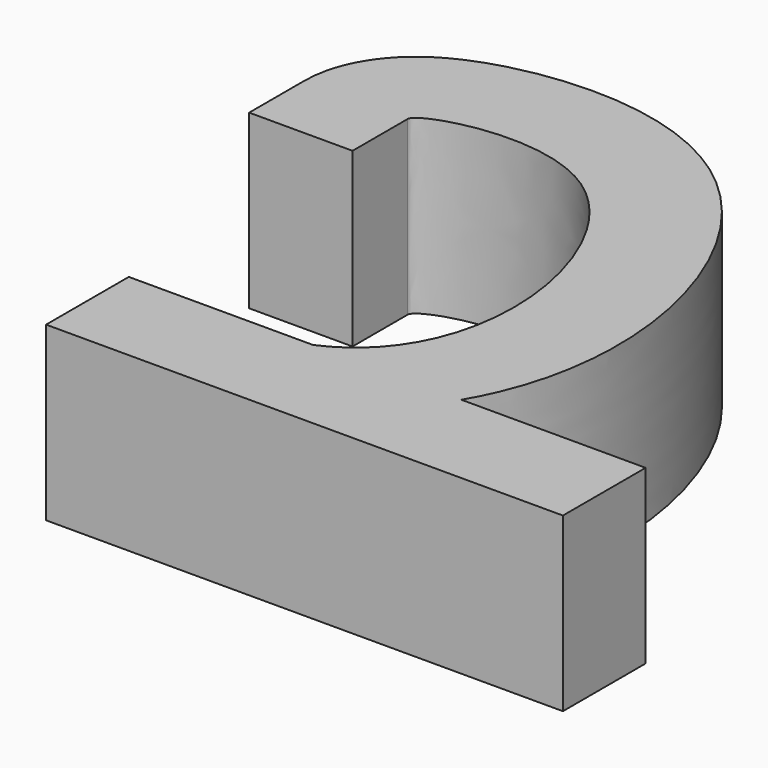
from build123d import *

# Parameters (mm, degrees)
F0_W     = 3
F0_H     = 2
F1_DEPTH = 5


# Not quite as in the source:
# - ends of sketch curves that miss each other by under 0.0002 mm in the source are joined
# - the dataset's text gives a spline's control points without its knots; the knots are read off the source's solid


with BuildPart() as f1:
    # F0 (on Top) → F1 (new body)
    with BuildSketch(Plane.XY):
        Polygon((0.2503667564, 0), (-5.0978784384, 0), (-5.0978784384, -3), (9.9021215616, -3), (9.9021215616, 0), (4.5538399041, 0), align=None)
        with BuildLine():
            add(Edge.make_bspline(
                [(-5.0038373292, 10), (-5.0038373292, 10.4105466628), (2.1157200772, 12.6615455049), (4.0203314378, 1.6529998477), (0.2503667564, 0)],
                knots=[0, 0, 0, 0, 0.4142686249, 1, 1, 1, 1], degree=3))
            Line((0.2503667564, 0), (4.5538399041, 0))
            add(Edge.make_bspline(
                [(-8.0038373298, 10), (-8.0038373298, 10.2787056237), (-7.9265937296, 10.7996899682), (-7.6932242014, 11.3893049019), (-7.4344399504, 11.8107970085), (-7.1058635967, 12.2133413532), (-6.7538412088, 12.5232161476), (-6.4054617225, 12.7628325838), (-6.0969380756, 12.93621453), (-5.8079542421, 13.0736567268), (-5.5258027553, 13.1889045793), (-5.1488196574, 13.3220823158), (-4.6640252083, 13.4592847565), (-4.0426527359, 13.5858120578), (-3.3762627135, 13.6713518347), (-2.6639349861, 13.7084653959), (-1.9073543006, 13.686135431), (-1.1101715023, 13.5900533961), (-0.2790603331, 13.4026671913), (0.5747150123, 13.1031110257), (1.2876198097, 12.743572644), (1.8463165534, 12.3791285027), (2.3650523455, 11.9843299327), (2.9469957376, 11.4415186656), (3.7495742807, 10.4950924187), (4.5420905535, 9.1980589469), (5.209598751, 7.5151054912), (5.6041511953, 5.7386647539), (5.7043043683, 3.8960335815), (5.4539395397, 2.0134312582), (4.9603909881, 0.7054202789), (4.5856072864, 0.0536222336), (4.5538399041, 0)],
                knots=[0, 0, 0, 0, 0.0078125, 0.015625, 0.0234375, 0.03125, 0.046875, 0.0625, 0.078125, 0.09375, 0.109375, 0.125, 0.15625, 0.1875, 0.21875, 0.25, 0.28125, 0.3125, 0.34375, 0.375, 0.40625, 0.421875, 0.4375, 0.46875, 0.5, 0.5625, 0.625, 0.6875, 0.75, 0.8125, 0.875, 0.8806276917, 0.8806276917, 0.8806276917, 0.8806276917], degree=3))
            Line((-8.0038373298, 10), (-5.0038373292, 10))
        make_face()
        with Locations((-6.5038373292, 9)):
            Rectangle(F0_W, F0_H)
    extrude(amount=F1_DEPTH)


solid = f1.part
